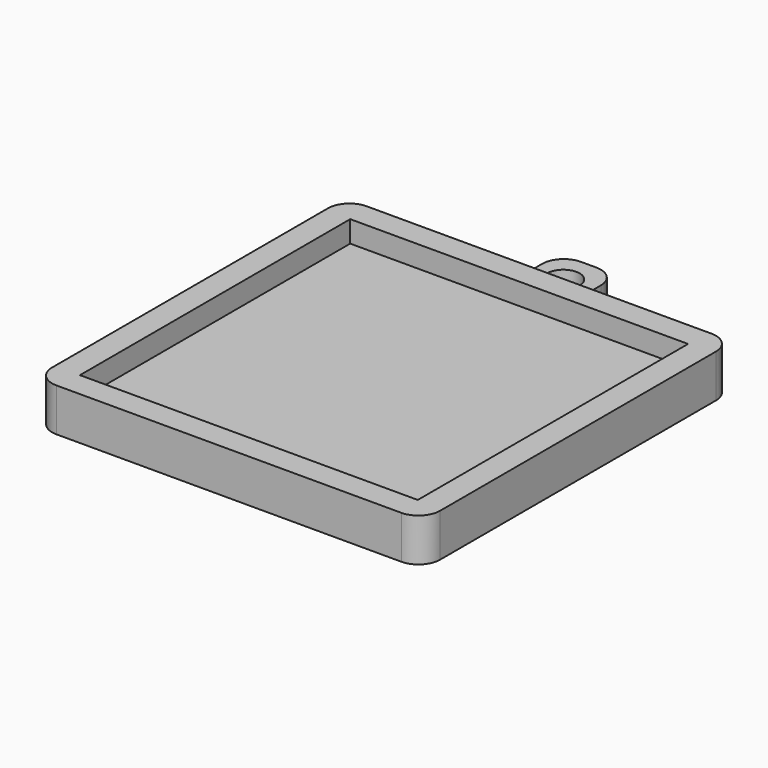
from build123d import *

# Parameters (mm, degrees)
F0_R     = 1.9252785304
F1_DEPTH = 2.54
F2_W     = 45.761115849
F2_H     = 45.761115849
F2_W_2   = 39.8514248748
F2_H_2   = 39.8514248748
F3_DEPTH = 2.54
F6_R     = 2.54


# Not quite as in the source:
# - a feature of the source that left no trace in its solid (it failed there, or was rolled back) is left out


with BuildPart() as f1:
    # F0 (on Top) → F1 (new body)
    with BuildSketch(Plane.XY):
        Polygon((-45.761115849, 0), (0, 0), (0, 45.761115849), (-19.5707920939, 45.761115849), (-19.5707920939, 53.2440654933), (-26.4781303704, 53.2440654933), (-26.4781303704, 45.761115849), (-45.761115849, 45.761115849), align=None)
        with Locations((-23.0244612321, 49.5025906712)):
            Circle(F0_R, mode=Mode.SUBTRACT)
    extrude(amount=F1_DEPTH)

    # F2 (on face) → F3 (join)
    with BuildSketch(Plane.XY.offset(2.54)):
        with Locations((-22.8805579245, 22.8805579245)):
            Rectangle(F2_W, F2_H)
        with Locations((-22.8805579245, 22.8805579245)):
            Rectangle(F2_W_2, F2_H_2, mode=Mode.SUBTRACT)
    extrude(amount=F3_DEPTH)

    # F6
    f6_edges = [f1.edges().sort_by_distance(p)[0] for p in [
        (-19.570792, 53.244065, 1.27),
        (-26.47813, 53.244065, 1.27),
        (0, 45.761116, 2.54),
        (0, 0, 2.54),
        (-45.761116, 0, 2.54),
        (-45.761116, 45.761116, 2.54),
    ]]
    fillet(f6_edges, radius=F6_R)


solid = f1.part
